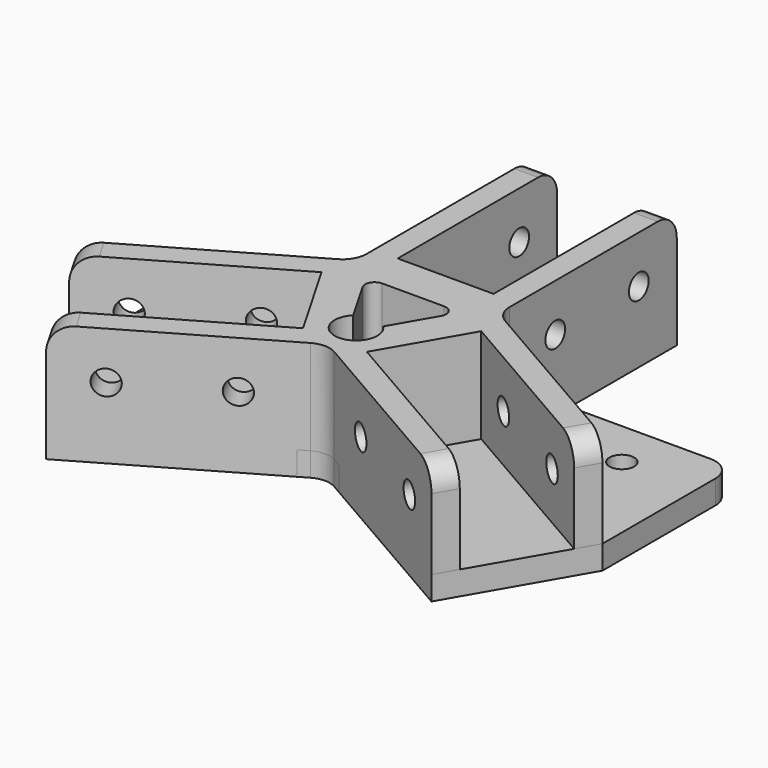
from build123d import *

# Parameters (mm, degrees)
F1_DEPTH    = 20
F2_R        = 2.6
F3_DEPTH    = 50.6016350946
F4_COUNT    = 3
F4_ANGLE    = 240
F6_DEPTH    = 5
F7_T1_DEPTH = 25
F10_DEPTH   = 5
F11_DEPTH   = 25.001
F12_R       = 2
F13_R       = 2.6
F14_DEPTH   = 25.001
F15_R       = 5
F16_R       = 4.5
F17_DEPTH   = 20


# Not quite as in the source:
# - a fillet or chamfer that OpenCascade refuses, or shapes differently, is made with other operations: its cross-section is extruded or revolved along the edge and cut away or added


with BuildPart() as f1:
    # F0 (on Top) → F1 (new body)
    with BuildSketch(Plane.XY):
        Polygon((43.0992290895, -36.5458269543), (6.7261621305, -15.5458269543), (16.8261621305, 1.9478862021), (53.1992290895, -19.0521137979), (55.6992290895, -14.7219867789), (14.8979589003, 8.8346375481), (0, 0), (-0.2020410997, -17.3193296462), (40.5992290895, -40.8759539732), align=None)
    extrude(amount=F1_DEPTH)

    # F2 (on face) → F3 (cut, through all)
    with BuildSketch(Plane(origin=(-7.55, -13.0769835971, 0), x_dir=(0.8660254038, -0.5, 0), z_dir=(-0.5, -0.8660254038, 0))):
        with Locations((45.5979407522, 10)):
            Circle(F2_R)
        with Locations((23.5979407522, 10)):
            Circle(F2_R)
    extrude(amount=-F3_DEPTH, mode=Mode.SUBTRACT)

    # F4: F1 ×3 about axis
    f4_axis = Axis((0, 0, 10), (0, 0, -1))


with BuildPart() as f1_1:
    add(f1.part)
    for i in range(1, F4_COUNT):
        add(f1.part.rotate(f4_axis, i * F4_ANGLE / (F4_COUNT - 1)))

    # F5 (on face) → F6 (join)
    with BuildSketch(Plane(origin=(0, 0, 0), x_dir=(1, 0, 0), z_dir=(0, 0, -1))):
        Polygon((0, 17.4359781295), (-40.5992290895, 40.8759539732), (-55.6992290895, 14.7219867789), (-15.1, -8.7179890648), (-15.1, -55.5979407522), (15.1, -55.5979407522), (15.1, -8.7179890648), (55.6992290895, 14.7219867789), (40.5992290895, 40.8759539732), align=None)
    extrude(amount=F6_DEPTH)

    # F7: fillet of radius 5 on 3 edges, made by hand

    # F7_s2 → F7_t1 (join)
    with BuildSketch(Plane.XY.offset(-5)):
        with BuildLine():
            ThreePointArc((2.5, -18.8792383324), (0, -18.2093653514), (-2.5, -18.8792383324))
            Line((-2.5, -18.8792383324), (-2.55, -18.7926357921))
            ThreePointArc((-2.55, -18.7926357921), (-1.299975, -18.0710489919), (-0.05, -17.3493755891))
            Line((-0.05, -17.3493755891), (0.05, -17.3493755891))
            ThreePointArc((0.05, -17.3493755891), (1.299975, -18.0710489919), (2.55, -18.7926357921))
            Line((2.55, -18.7926357921), (2.5, -18.8792383324))
        make_face()
        with BuildLine():
            ThreePointArc((15.0999, 11.6046826757), (15.7697729811, 9.1046826757), (17.5999, 7.2745556568))
            Line((17.5999, 7.2745556568), (17.5499, 7.1879531164))
            ThreePointArc((17.5499, 7.1879531164), (16.299975, 7.9097131217), (15.05, 8.6313865244))
            Line((15.05, 8.6313865244), (15, 8.7179890648))
            ThreePointArc((15, 8.7179890648), (15, 10.1613358702), (14.9999, 11.6046826757))
            Line((14.9999, 11.6046826757), (15.0999, 11.6046826757))
        make_face()
        with BuildLine():
            ThreePointArc((-17.5999, 7.2745556568), (-15.7697729811, 9.1046826757), (-15.0999, 11.6046826757))
            Line((-15.0999, 11.6046826757), (-14.9999, 11.6046826757))
            ThreePointArc((-14.9999, 11.6046826757), (-15, 10.1613358702), (-15, 8.7179890648))
            Line((-15, 8.7179890648), (-15.05, 8.6313865244))
            ThreePointArc((-15.05, 8.6313865244), (-16.299975, 7.9097131217), (-17.5499, 7.1879531164))
            Line((-17.5499, 7.1879531164), (-17.5999, 7.2745556568))
        make_face()
    extrude(amount=F7_T1_DEPTH)

    # F9 (on face) → F10 (join)
    with BuildSketch(Plane(origin=(0, 0, -5), x_dir=(1, 0, 0), z_dir=(0, 0, -1))):
        with BuildLine():
            Line((-55.6992290895, 14.7219867789), (-55.6992290895, -20))
            Line((-55.6992290895, -20), (55.6992290895, -20))
            Line((55.6992290895, -20), (55.6992290895, 14.7219867789))
            Line((55.6992290895, 14.7219867789), (52.6519667355, 20))
            Line((52.6519667355, 20), (4.4410161514, 20))
            Line((4.4410161514, 20), (2.5, 18.8793538025))
            ThreePointArc((2.5, 18.8793538025), (0, 18.2094808214), (-2.5, 18.8793538025))
            Line((-2.5, 18.8793538025), (-4.4410161514, 20))
            Line((-4.4410161514, 20), (-52.6519667355, 20))
            Line((-52.6519667355, 20), (-55.6992290895, 14.7219867789))
        make_face()
    extrude(amount=-F10_DEPTH)

    # F8 (on face) → F11 (cut, through all)
    with BuildSketch(Plane.XY.offset(20)):
        Polygon((10, 5.0614941438), (-10, 5.0614941438), (0, -12.2590139319), align=None)
    extrude(amount=-F11_DEPTH, mode=Mode.SUBTRACT)

    # F12
    f12_edges = [f1_1.edges().sort_by_distance(p)[0] for p in [
        (10, 5.061494, 7.5),
        (-10, 5.061494, 7.5),
        (0, -12.259014, 7.5),
    ]]
    fillet(f12_edges, radius=F12_R)

    # F13 (on face) → F14 (cut, through all)
    with BuildSketch(Plane(origin=(0, 0, -5), x_dir=(1, 0, 0), z_dir=(0, 0, -1))):
        with Locations((-40, -10)):
            Circle(F13_R)
        with Locations((40, -10)):
            Circle(F13_R)
        with Locations((0, 10)):
            Circle(F13_R)
    extrude(amount=-F14_DEPTH, mode=Mode.SUBTRACT)

    # F15
    f15_edges = [f1_1.edges().sort_by_distance(p)[0] for p in [
        (-15.1, 20, -2.5),
        (15.1, 20, -2.5),
        (55.699229, 20, -2.5),
        (-55.699229, 20, -2.5),
        (-12.6, 55.597941, 20),
        (12.6, 55.597941, 20),
        (-54.449229, -16.88705, 20),
        (-41.849229, -38.71089, 20),
        (54.449229, -16.88705, 20),
        (41.849229, -38.71089, 20),
    ]]
    fillet(f15_edges, radius=F15_R)

    # F16 (on face) → F17 (cut)
    with BuildSketch(Plane.XY.offset(20)):
        with Locations((0, -10)):
            Circle(F16_R)
    extrude(amount=-F17_DEPTH, mode=Mode.SUBTRACT)


solid = f1_1.part
